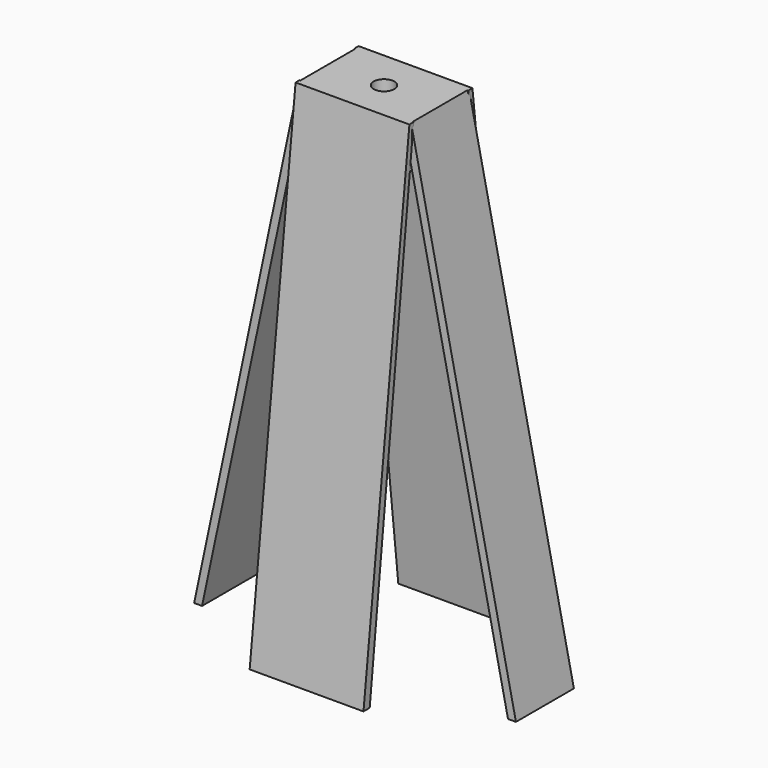
from build123d import *

# Parameters (mm, degrees)
F0_W           = 279.4
F0_H           = 190.5
F1_DEPTH       = 101.6
F3_DEPTH       = 279.401
F5_DEPTH       = 190.501
F7_DEPTH       = 139.7
F7_DEPTH_BACK  = 139.7
F8_R           = 25.4
F9_DEPTH       = 1211.0351297934
F11_DEPTH      = 88.9
F11_DEPTH_BACK = 88.9
F12_DEPTH      = 25
F12_DEPTH_BACK = 25


# Not quite as in the source:
# - a pattern or mirror of a feature is missing from the dataset's text; its kind, count and spacing are read off the source's solid


with BuildPart() as f1:
    # F0 (on Top) → F1 (new body)
    with BuildSketch(Plane.XY):
        Rectangle(F0_W, F0_H)
    extrude(amount=-F1_DEPTH)

    # F2 (on face) → F3 (cut, through all)
    with BuildSketch(Plane.YZ.offset(139.7)):
        Polygon((-95.25, -101.6), (-83.9622399803, 0), (-95.25, 0), align=None)
    extrude(amount=-F3_DEPTH, mode=Mode.SUBTRACT)

    # F4 (on face) → F5 (cut, through all)
    with BuildSketch(Plane(origin=(0, 95.25, 0), x_dir=(-1, 0, 0), z_dir=(0, 1, 0))):
        Polygon((-139.7, -101.6), (-118.1042533343, 0), (-139.7, 0), align=None)
    f5 = extrude(amount=-F5_DEPTH, mode=Mode.SUBTRACT)

    # F5_copies: F5 across plane
    add(f5.mirror(Plane(origin=(0, 0, 0), x_dir=(0, 0, -1), z_dir=(-1, 0, 0))), mode=Mode.SUBTRACT)

    # F6 (on Right) → F7 (join, two sides)
    with BuildSketch(Plane.YZ) as f7_sk:
        Polygon((-218.5081320352, -1211.0341297934), (-95.25, -101.6), (-83.9622399803, 0), (-96.6859329486, 0), (-237.5581320352, -1211.0341297934), align=None)
    f7 = extrude(amount=F7_DEPTH) + extrude(f7_sk.sketch, amount=-F7_DEPTH_BACK)

    # F7_copies: F7 across plane
    add(f7.mirror(Plane.ZX))

    # F8 (on face) → F9 (cut, through all)
    with BuildSketch(Plane.XY):
        Circle(F8_R)
    extrude(amount=-F9_DEPTH, mode=Mode.SUBTRACT)

    # F10 (on Front) → F11 (join, two sides)
    with BuildSketch(Plane.XZ) as f11_sk:
        Polygon((-139.7, -9.9745607326), (-139.7, -101.6), (-118.1042533343, 0), (-137.5798416665, 0), align=None)
        Polygon((-375.5175040283, -1211.0341297934), (-139.7, -101.6), (-139.7, -9.9745607326), (-394.9930923604, -1211.0341297934), align=None)
    f11 = extrude(amount=F11_DEPTH) + extrude(f11_sk.sketch, amount=-F11_DEPTH_BACK)

    # F11_copies: F11 across plane
    add(f11.mirror(Plane(origin=(0, 0, 0), x_dir=(0, 0, 1), z_dir=(1, 0, 0))))

    # F10 (on Front) → F12 (join, two sides)
    with BuildSketch(Plane.XZ) as f12_sk:
        Polygon((-375.5175040283, -1211.0341297934), (-139.7, -101.6), (-139.7, -9.9745607326), (-394.9930923604, -1211.0341297934), align=None)
        Polygon((-139.7, -9.9745607326), (-139.7, -101.6), (-118.1042533343, 0), (-137.5798416665, 0), align=None)
    extrude(amount=F12_DEPTH)
    extrude(f12_sk.sketch, amount=-F12_DEPTH_BACK)


solid = f1.part
